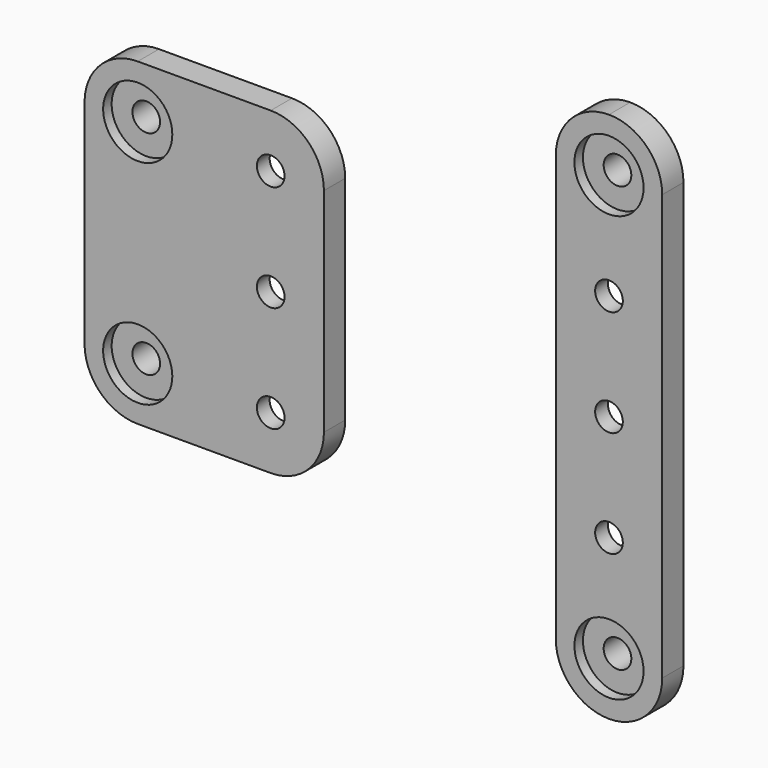
from build123d import *

# Parameters (mm, degrees)
F0_W             = 20
F0_H             = 100
F0_R             = 3.6
F1_DEPTH         = 5
F0_W_2           = 45
F0_H_2           = 60
F2_DEPTH         = 6
F4_D             = 5.2
F4_CBORE_D       = 13
F4_CBORE_DEPTH   = 2
F4_2_D           = 5.2
F4_2_CBORE_D     = 13
F4_2_CBORE_DEPTH = 2
F5_R             = 9.99999
F5_2_R           = 9.99999
F6_D             = 5.2
F6_CBORE_D       = 13
F6_CBORE_DEPTH   = 2
F6_2_D           = 5.2
F6_2_CBORE_D     = 13
F6_2_CBORE_DEPTH = 2


# Not quite as in the source:
# - a fillet or chamfer is up to 0.001 mm smaller than in the source, because OpenCascade refuses the exact size


with BuildPart() as f1:
    # F0 (on Front) → F1 (new body)
    with BuildSketch(Plane.XZ):
        with Locations((41.227266416, 0)):
            Rectangle(F0_W, F0_H)
        with Locations((41.227266416, -40)):
            Circle(F0_R, mode=Mode.SUBTRACT)
        with Locations((41.227266416, 40)):
            Circle(F0_R, mode=Mode.SUBTRACT)
        with Locations((41.227266416, -40)):
            Circle(F0_R)
        with Locations((41.227266416, 40)):
            Circle(F0_R)
    extrude(amount=F1_DEPTH)

    # F0 (on Front) → F2, piece 2 (join)
    with BuildSketch(Plane.XZ):
        with Locations((41.227266416, 40)):
            Circle(F0_R)
        with Locations((41.227266416, -40)):
            Circle(F0_R)
    extrude(amount=-F2_DEPTH)

    # F4 (through all)
    with Locations(Plane(origin=(0, 0, 0), x_dir=(1, 0, 0), z_dir=(0, 1, 0))):
        with Locations((41.227266416, -20), (41.227266416, 0), (41.227266416, 20), (-22.3634822667, -20), (-22.3634822667, 0), (-22.3634822667, 20)):
            CounterBoreHole(F4_D / 2, F4_CBORE_D / 2, F4_CBORE_DEPTH)

    # F5 (radius 10 in the source; OpenCascade refuses exactly that, so slightly less here)
    f5_edges = [f1.edges().sort_by_distance(p)[0] for p in [
        (31.227266, -2.5, 50),
        (51.227266, -2.5, 50),
        (31.227266, -2.5, -50),
        (51.227266, -2.5, -50),
    ]]
    fillet(f5_edges, radius=F5_R)

    # F6 (through all)
    with Locations(Plane.XZ.offset(5)):
        with Locations((41.227266416, 40), (41.227266416, -40), (-47.3634822667, 20), (-47.3634822667, -20)):
            CounterBoreHole(F6_D / 2, F6_CBORE_D / 2, F6_CBORE_DEPTH)


with BuildPart() as f1b:
    # F0 (on Front) → F1, piece 2 (new body)
    with BuildSketch(Plane.XZ):
        with Locations((-34.8634822667, 0)):
            Rectangle(F0_W_2, F0_H_2)
        with Locations((-47.3634822667, -20)):
            Circle(F0_R, mode=Mode.SUBTRACT)
        with Locations((-47.3634822667, 20)):
            Circle(F0_R, mode=Mode.SUBTRACT)
        with Locations((-47.3634822667, 20)):
            Circle(F0_R)
        with Locations((-47.3634822667, -20)):
            Circle(F0_R)
    extrude(amount=F1_DEPTH)

    # F0 (on Front) → F2 (join)
    with BuildSketch(Plane.XZ):
        with Locations((-47.3634822667, 20)):
            Circle(F0_R)
        with Locations((-47.3634822667, -20)):
            Circle(F0_R)
    extrude(amount=-F2_DEPTH)

    # F4#2 (through all)
    with Locations(Plane(origin=(0, 0, 0), x_dir=(1, 0, 0), z_dir=(0, 1, 0))):
        with Locations((41.227266416, -20), (41.227266416, 0), (41.227266416, 20), (-22.3634822667, -20), (-22.3634822667, 0), (-22.3634822667, 20)):
            CounterBoreHole(F4_2_D / 2, F4_2_CBORE_D / 2, F4_2_CBORE_DEPTH)

    # F5#2 (radius 10 in the source; OpenCascade refuses exactly that, so slightly less here)
    f5_2_edges = [f1b.edges().sort_by_distance(p)[0] for p in [
        (-57.363482, -2.5, 30),
        (-57.363482, -2.5, -30),
        (-12.363482, -2.5, -30),
        (-12.363482, -2.5, 30),
    ]]
    fillet(f5_2_edges, radius=F5_2_R)

    # F6#2 (through all)
    with Locations(Plane.XZ.offset(5)):
        with Locations((41.227266416, 40), (41.227266416, -40), (-47.3634822667, 20), (-47.3634822667, -20)):
            CounterBoreHole(F6_2_D / 2, F6_2_CBORE_D / 2, F6_2_CBORE_DEPTH)


solid = Compound([f1.part, f1b.part])
